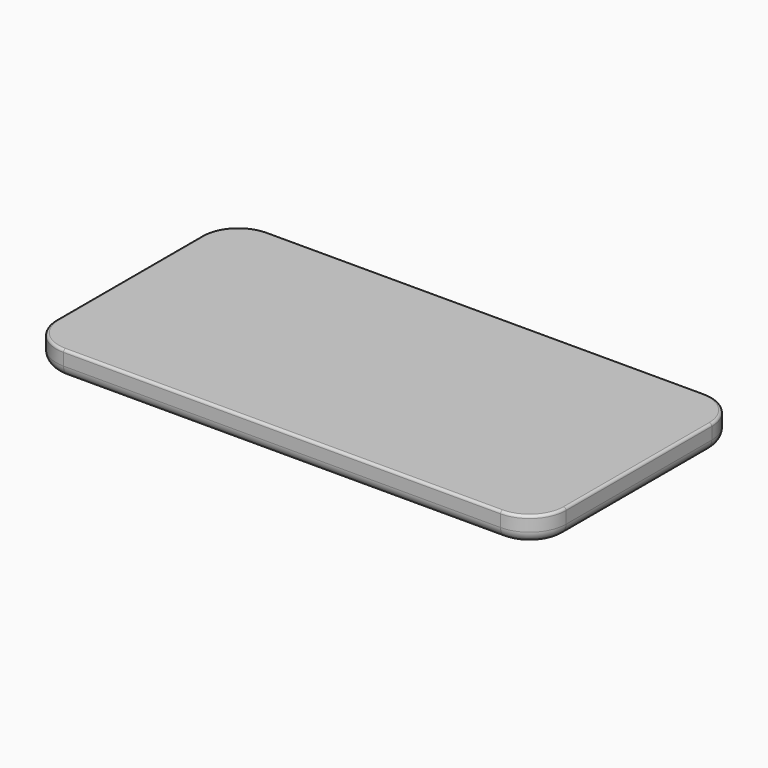
from build123d import *

# Parameters (mm, degrees)
F0_W         = 140
F0_H         = 70
F1_DEPTH     = 7
F2_R         = 10
F3_R         = 0.7
F4_R         = 3
F6_DEPTH     = 1
F7_R         = 2
F8_T1_DEPTH  = 8
F8_T3_DEPTH  = 8
F8_T6_ANGLE  = 90
F8_T8_ANGLE  = 90
F8_T10_ANGLE = 90
F8_T12_ANGLE = 90
F9_DEPTH     = 0.5
F10_R        = 1.5
F11_DEPTH    = 0.1


# Not quite as in the source:
# - a fillet or chamfer that OpenCascade refuses, or shapes differently, is made with other operations: its cross-section is extruded or revolved along the edge and cut away or added


with BuildPart() as f1:
    # F0 (on Top) → F1 (new body)
    with BuildSketch(Plane.XY):
        with Locations((18.6064650118, 35)):
            Rectangle(F0_W, F0_H)
    extrude(amount=F1_DEPTH)

    # F2
    f2_edges = [f1.edges().sort_by_distance(p)[0] for p in [
        (88.606465, 70, 3.5),
        (88.606465, 0, 3.5),
        (-51.393535, 0, 3.5),
        (-51.393535, 70, 3.5),
    ]]
    fillet(f2_edges, radius=F2_R)

    # F3
    f3_edges = [f1.edges().sort_by_distance(p)[0] for p in [
        (18.606465, 0, 7),
        (88.606465, 35, 7),
        (85.677533, 2.928932, 7),
        (85.677533, 67.071068, 7),
        (18.606465, 70, 7),
        (-48.464603, 2.928932, 7),
        (-48.464603, 67.071068, 7),
        (-51.393535, 35, 7),
    ]]
    fillet(f3_edges, radius=F3_R)

    # F4
    f4_edges = [f1.edges().sort_by_distance(p)[0] for p in [
        (18.606465, 0, 0),
        (88.606465, 35, 0),
        (85.677533, 2.928932, 0),
        (85.677533, 67.071068, 0),
        (18.606465, 70, 0),
        (-48.464603, 2.928932, 0),
        (-48.464603, 67.071068, 0),
        (-51.393535, 35, 0),
    ]]
    fillet(f4_edges, radius=F4_R)

    # F5 (on face) → F6 (join)
    with BuildSketch(Plane(origin=(0, 0, 0), x_dir=(1, 0, 0), z_dir=(0, 0, -1))):
        Polygon((78.6064650118, -41), (78.6064650118, -35), (78.6064650118, -29), (66.6064650118, -29), (66.6064650118, -41), align=None)
    extrude(amount=F6_DEPTH)

    # F7
    f7_edges = [f1.edges().sort_by_distance(p)[0] for p in [
        (66.606465, 41, -0.5),
        (66.606465, 29, -0.5),
        (78.606465, 29, -0.5),
        (78.606465, 41, -0.5),
    ]]
    fillet(f7_edges, radius=F7_R)

    # F8: fillet of radius 2 on 1 edges, made by hand

    # F8_s2 → F8_t1 (cut)
    with BuildSketch(Plane.YZ.offset(68.6064650118)):
        with BuildLine():
            ThreePointArc((41, 0), (40.2679491924, -0.7320508076), (39.2679491924, -1))
            Line((39.2679491924, -1), (41, -1))
            Line((41, -1), (41, 0))
        make_face()
        with BuildLine():
            ThreePointArc((29, 0), (29.7320508076, -0.7320508076), (30.7320508076, -1))
            Line((30.7320508076, -1), (29, -1))
            Line((29, -1), (29, 0))
        make_face()
    extrude(amount=F8_T1_DEPTH, mode=Mode.SUBTRACT)

    # F8_s4 → F8_t3 (cut)
    with BuildSketch(Plane.XZ.offset(-39)):
        with BuildLine():
            ThreePointArc((78.6064650118, 0), (77.8744142043, -0.7320508076), (76.8744142043, -1))
            Line((76.8744142043, -1), (78.6064650118, -1))
            Line((78.6064650118, -1), (78.6064650118, 0))
        make_face()
        with BuildLine():
            ThreePointArc((66.6064650118, 0), (67.3385158194, -0.7320508076), (68.3385158194, -1))
            Line((68.3385158194, -1), (66.6064650118, -1))
            Line((66.6064650118, -1), (66.6064650118, 0))
        make_face()
    extrude(amount=F8_T3_DEPTH, mode=Mode.SUBTRACT)

    # F8_s5 → F8_t6 (revolve, cut)
    with BuildSketch(Plane.YZ.offset(68.6064650118)):
        with BuildLine():
            ThreePointArc((41, 0), (40.2679491924, -0.7320508076), (39.2679491924, -1))
            Line((39.2679491924, -1), (41, -1))
            Line((41, -1), (41, 0))
        make_face()
    revolve(axis=Axis((68.6064650118, 39, -1), (0, 0, 1)), revolution_arc=F8_T6_ANGLE, mode=Mode.SUBTRACT)

    # F8_s7 → F8_t8 (revolve, cut)
    with BuildSketch(Plane.YZ.offset(76.6064650118)):
        with BuildLine():
            ThreePointArc((41, 0), (40.2679491924, -0.7320508076), (39.2679491924, -1))
            Line((39.2679491924, -1), (41, -1))
            Line((41, -1), (41, 0))
        make_face()
    revolve(axis=Axis((76.6064650118, 39, -1), (0, 0, -1)), revolution_arc=F8_T8_ANGLE, mode=Mode.SUBTRACT)

    # F8_s9 → F8_t10 (revolve, cut)
    with BuildSketch(Plane.YZ.offset(76.6064650118)):
        with BuildLine():
            ThreePointArc((29, 0), (29.7320508076, -0.7320508076), (30.7320508076, -1))
            Line((30.7320508076, -1), (29, -1))
            Line((29, -1), (29, 0))
        make_face()
    revolve(axis=Axis((76.6064650118, 31, -1), (0, 0, 1)), revolution_arc=F8_T10_ANGLE, mode=Mode.SUBTRACT)

    # F8_s11 → F8_t12 (revolve, cut)
    with BuildSketch(Plane.XZ.offset(-31)):
        with BuildLine():
            ThreePointArc((66.6064650118, 0), (67.3385158194, -0.7320508076), (68.3385158194, -1))
            Line((68.3385158194, -1), (66.6064650118, -1))
            Line((66.6064650118, -1), (66.6064650118, 0))
        make_face()
    revolve(axis=Axis((68.6064650118, 31, -1), (0, 0, 1)), revolution_arc=F8_T12_ANGLE, mode=Mode.SUBTRACT)

    # F9 (cut): faces of the model
    f9_faces = [f1.faces().sort_by_distance(p)[0] for p in [
        (72.6064650118, 35, -1),
        (17.7021104435, 35, 0),
    ]]
    extrude(f9_faces, amount=F9_DEPTH, mode=Mode.SUBTRACT)

    # F10 (on face) → F11 (cut)
    with BuildSketch(Plane(origin=(0, 0, -1), x_dir=(1, 0, 0), z_dir=(0, 0, -1))):
        with Locations((72.6282298565, -35)):
            Circle(F10_R)
    extrude(amount=-F11_DEPTH, mode=Mode.SUBTRACT)


solid = f1.part
